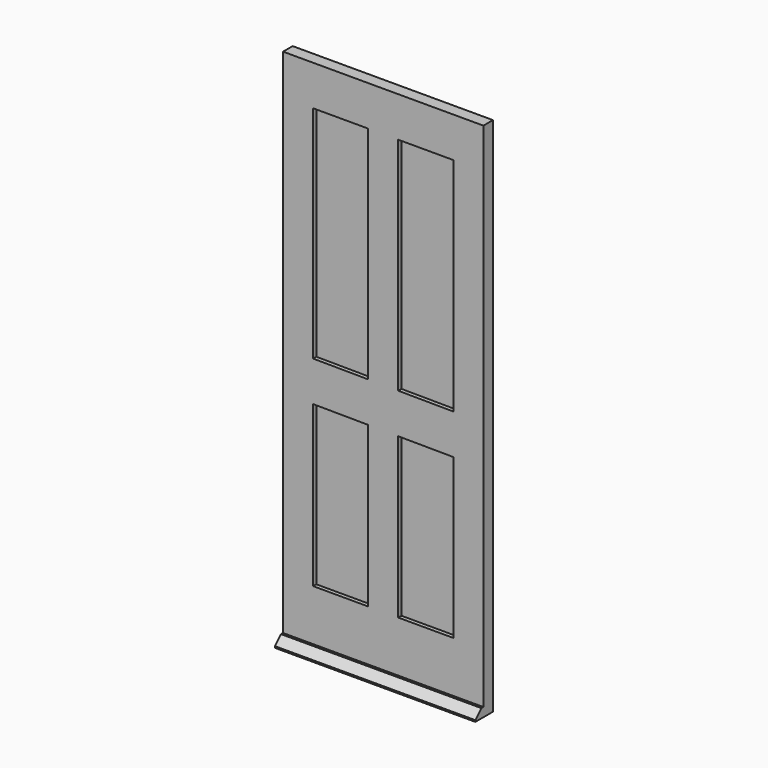
from build123d import *

# Parameters (mm, degrees)
F1_DEPTH      = 0.4
F1_DEPTH_BACK = 0.4
F0_W          = 6
F0_H          = 8
F0_H_2        = 12
F2_DEPTH      = 1.2
F2_DEPTH_BACK = 1.2
F3_W          = 40
F3_H          = 1.8093388975
F4_DEPTH      = 2
F5_SIZE       = 1.5


# Not quite as in the source:
# - ends of sketch curves that miss each other by under 0.0002 mm in the source are joined


with BuildPart() as f1:
    # F0 (on Front) → F1 (new body, two sides)
    with BuildSketch(Plane.XZ) as f1_sk:
        Polygon((-3, 44), (-14, 44), (-14, 0), (-3, -0.0798979561), align=None)
    extrude(amount=F1_DEPTH)
    extrude(f1_sk.sketch, amount=-F1_DEPTH_BACK)


with BuildPart() as f1b:
    # F0 (on Front) → F1, piece 2 (new body, two sides)
    with BuildSketch(Plane.XZ) as f1_2_sk:
        Polygon((14, -0.2033766155), (14, 44), (3, 44), (3, -0.1234786594), align=None)
    extrude(amount=F1_DEPTH)
    extrude(f1_2_sk.sketch, amount=-F1_DEPTH_BACK)


with BuildPart() as f1c:
    # F0 (on Front) → F1, piece 3 (new body, two sides)
    with BuildSketch(Plane.XZ) as f1_3_sk:
        Polygon((-3, -8.0801089842), (-14.0000014294, -8.0002110177), (-14, -40), (-3, -40), align=None)
    extrude(amount=F1_DEPTH)
    extrude(f1_3_sk.sketch, amount=-F1_DEPTH_BACK)


with BuildPart() as f1d:
    # F0 (on Front) → F1, piece 4 (new body, two sides)
    with BuildSketch(Plane.XZ) as f1_4_sk:
        Polygon((3, -40), (14, -40), (14, -8.2035876436), (3, -8.1236896875), align=None)
    extrude(amount=F1_DEPTH)
    extrude(f1_4_sk.sketch, amount=-F1_DEPTH_BACK)


with BuildPart() as f2:
    # F0 (on Front) → F2 (new body, two sides)
    with BuildSketch(Plane.XZ) as f2_sk:
        with Locations((-17, 48)):
            Rectangle(F0_W, F0_H)
        Polygon((14, 44), (14, 52), (-14, 52), (-14, 44), (-3, 44), (3, 44), align=None)
        with Locations((17, 48)):
            Rectangle(F0_W, F0_H)
        Polygon((20, -40), (20, 44), (14, 44), (14, -0.2033766155), (14, -8.2035876436), (14, -40), align=None)
        Polygon((3, -0.1234786594), (3, 44), (-3, 44), (-3, -0.0798979561), align=None)
        Polygon((-14, 0), (-14, 44), (-20, 44), (-20, -40), (-14, -40), (-14, -8.0002110177), align=None)
        Polygon((-3, -0.0798979561), (-14, 0), (-14, -8.0002110177), (-3, -8.0801089842), align=None)
        Polygon((3, -8.1236896875), (3, -0.1234786594), (-3, -0.0798979561), (-3, -8.0801089842), align=None)
        Polygon((14, -8.2035876436), (14, -0.2033766155), (3, -0.1234786594), (3, -8.1236896875), align=None)
        Polygon((-3, -40), (3, -40), (3, -8.1236896875), (-3, -8.0801089842), align=None)
        with Locations((-17, -46)):
            Rectangle(F0_W, F0_H_2)
        Polygon((14, -52), (14, -40), (3, -40), (-3, -40), (-14, -40), (-14, -52), align=None)
        with Locations((17, -46)):
            Rectangle(F0_W, F0_H_2)
    extrude(amount=F2_DEPTH)
    extrude(f2_sk.sketch, amount=-F2_DEPTH_BACK)

    # F3 (on face) → F4 (join)
    with BuildSketch(Plane.XZ.offset(1.2)):
        with Locations((0, -51.0953305513)):
            Rectangle(F3_W, F3_H)
    extrude(amount=F4_DEPTH)

    # F5
    f5_edges = [f2.edges().sort_by_distance(p)[0] for p in [
        (0, -3.2, -50.190661),
    ]]
    chamfer(f5_edges, length=F5_SIZE)


solid = Compound([f1.part, f1b.part, f1c.part, f1d.part, f2.part])
